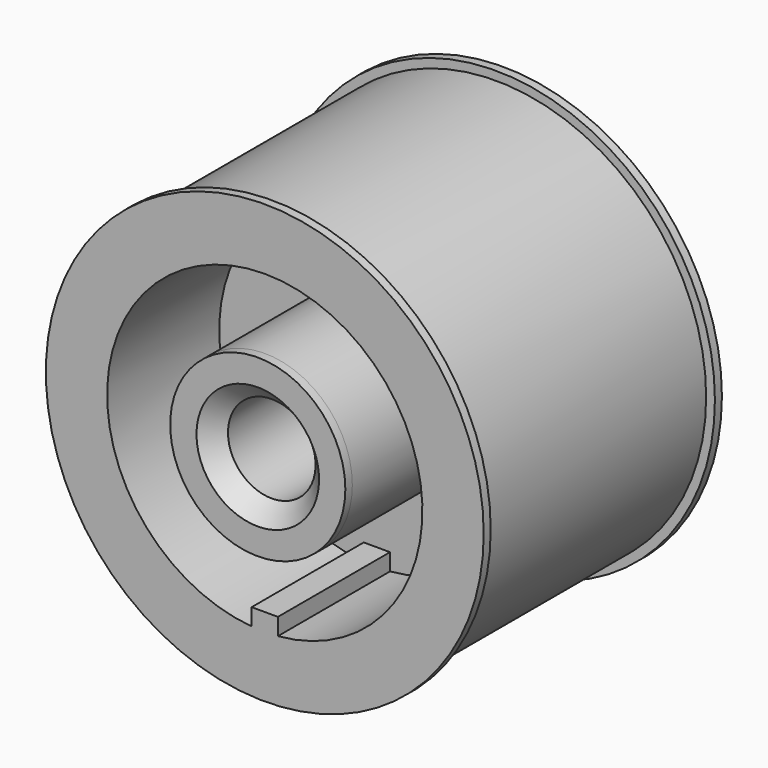
from build123d import *
from build123d import SkipClean  # not in build123d's __all__

# Parameters (mm, degrees)
F0_R         = 12.5
F1_DEPTH     = 17
F2_W         = 1.5
F2_H         = 16
F4_R         = 2.5
F5_DEPTH     = 17.001
F6_R         = 9
F6_R_2       = 5
F7_DEPTH     = 8
F8_W         = 4.9303688211
F8_H         = 2
F9_DEPTH     = 0.5
F10_R        = 5
F11_DEPTH    = 8
F12_DEPTH    = 0.5
F13_DEPTH    = 0.5
F14_T4_ANGLE = 359.64


# Not quite as in the source:
# - a fillet or chamfer that OpenCascade refuses, or shapes differently, is made with other operations: its cross-section is extruded or revolved along the edge and cut away or added
# - after a boolean that leaves OpenCascade's solid faulty, fix() repairs it


with BuildPart() as f1:
    # F0 (on Front) → F1 (new body)
    with BuildSketch(Plane.XZ):
        Circle(F0_R)
    extrude(amount=F1_DEPTH)

    # F2 (on Top) → F3 (revolve, cut)
    with BuildSketch(Plane.XY):
        with Locations((-12.75, -8.5)):
            Rectangle(F2_W, F2_H)
    revolve(axis=Axis((0, -8.2131072704, 0), (0, -1, 0)), mode=Mode.SUBTRACT)

    # F4 (on face) → F5 (cut, through all)
    with BuildSketch(Plane(origin=(0, 0, 0), x_dir=(-1, 0, 0), z_dir=(0, 1, 0))):
        Circle(F4_R)
    extrude(amount=-F5_DEPTH, mode=Mode.SUBTRACT)

    # F6 (on face) → F7 (cut)
    with BuildSketch(Plane(origin=(0, 0, 0), x_dir=(-1, 0, 0), z_dir=(0, 1, 0))):
        Circle(F6_R)
        Circle(F6_R_2, mode=Mode.SUBTRACT)
    extrude(amount=-F7_DEPTH, mode=Mode.SUBTRACT)

    # F8 (on face) → F9 (cut)
    with BuildSketch(Plane(origin=(0, 0, 0), x_dir=(-1, 0, 0), z_dir=(0, 1, 0))):
        with Locations((-3.8676508702, 0)):
            Rectangle(F8_W, F8_H)
    extrude(amount=-F9_DEPTH, mode=Mode.SUBTRACT)

    # F10 (on face) → F11 (cut)
    with BuildSketch(Plane.XZ.offset(17)):
        with BuildLine():
            Line((0.75, -8), (0.75, -8.9686955573))
            ThreePointArc((0.75, -8.9686955573), (0, 9), (-0.75, -8.9686955573))
            Line((-0.75, -8.9686955573), (-0.75, -8))
            Line((-0.75, -8), (0.75, -8))
        make_face()
        Circle(F10_R, mode=Mode.SUBTRACT)
    extrude(amount=-F11_DEPTH, mode=Mode.SUBTRACT)

    # F12 (add): a face of the model
    f12_faces = [f1.faces().sort_by_distance(p)[0] for p in [
        (-0.4884023099, 0, 4.8346844466),
    ]]
    with SkipClean():  # cleaning this boolean's faces spoils the solid; the shape is the same uncleaned
        extrude(f12_faces, amount=F12_DEPTH)

    # F13 (add): a face of the model
    f13_faces = [f1.faces().sort_by_distance(p)[0] for p in [
        (-4.8585786438, -17, 0),
    ]]
    extrude(f13_faces, amount=F13_DEPTH)

    add(f1.part.fix(), mode=Mode.REPLACE)

    # F14: chamfer of 1 on 2 edges, made by hand

    # F14_s1 → F14_t2 (revolve, cut)
    with BuildSketch(Plane.XY):
        Polygon((-2.5, -16.5), (-3.5, -17.5), (-2.5, -17.5), align=None)
    revolve(axis=Axis((0, -17.5, 0), (0, 1, 0)), mode=Mode.SUBTRACT)

    # F14_s3 → F14_t4 (revolve, cut)
    with BuildSketch(Plane(origin=(0, 0, 0), x_dir=(0, 1, 0), z_dir=(0.0031415875, 0, 0.9999950652))):
        Polygon((0.5, -3.5), (-0.5, -2.5), (0.5, -2.5), align=None)
    revolve(axis=Axis((0, 0.5, 0), (0, 1, 0)), revolution_arc=F14_T4_ANGLE, mode=Mode.SUBTRACT)


solid = f1.part
